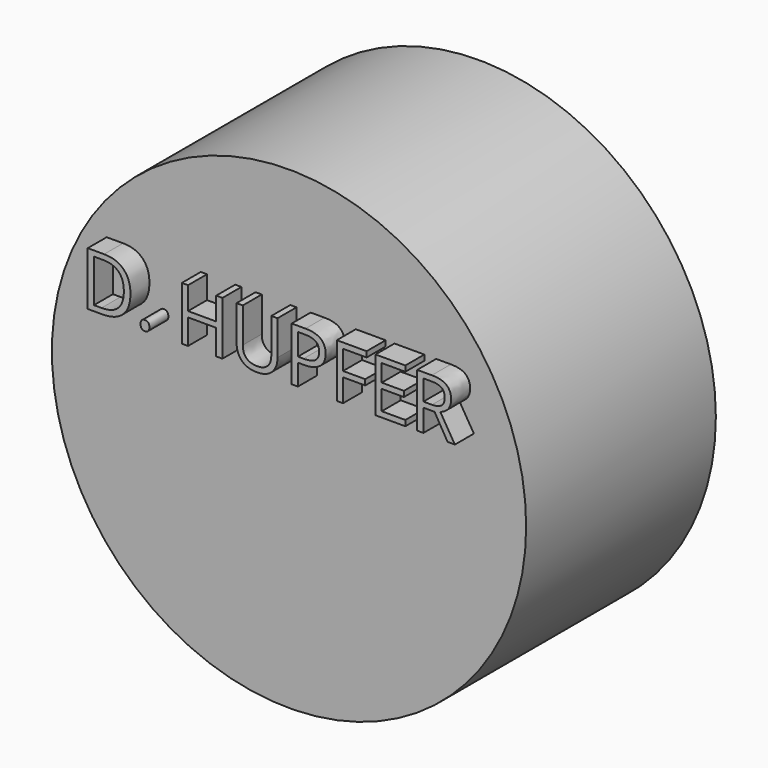
from build123d import *

# Parameters (mm, degrees)
F0_R         = 12.7
F1_DEPTH     = 12.7
F2_TEXT_SIZE = 4.0150663785
F3_DEPTH     = 1.27


# Not quite as in the source:
# - Text() gives the source's letters only with a copy of the font that has no kerning and outlines rounded to 1/6400 em; it was checked with that copy


with BuildPart() as f1:
    # F0 (on Front) → F1 (new body)
    with BuildSketch(Plane.XZ):
        with Locations((34.7411893308, 37.1474996209)):
            Circle(F0_R)
    extrude(amount=F1_DEPTH)

    # F2 (on face) → F3 (join)
    with BuildSketch(Plane.XZ.offset(12.7)):
        with Locations((24.5811893308, 40.6066518284)):
            Text('D. HUPFER', F2_TEXT_SIZE, font='Open Sans', text_align=(TextAlign.LEFT, TextAlign.BOTTOM))
    extrude(amount=F3_DEPTH)


solid = f1.part
